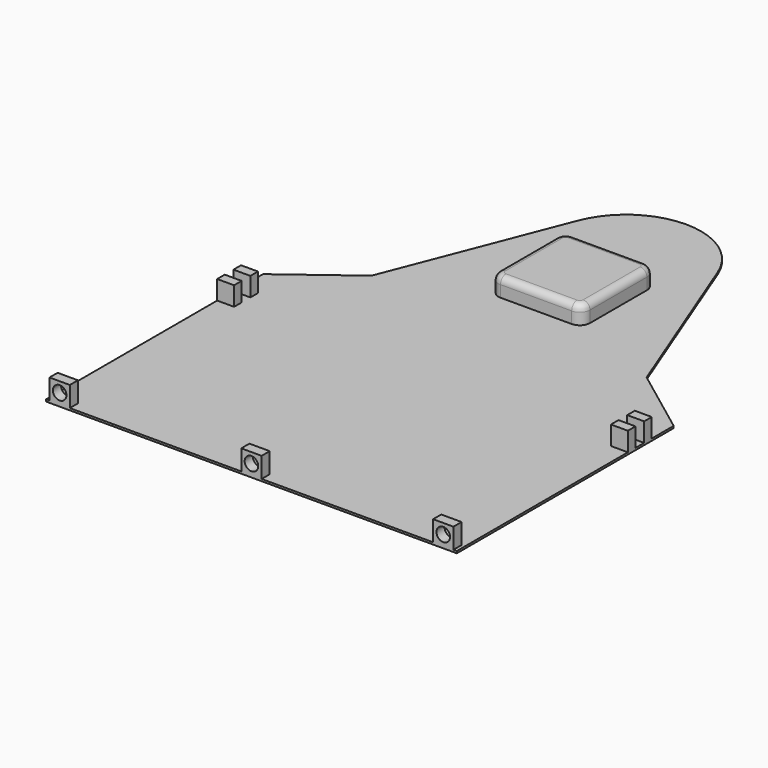
from build123d import *

# Parameters (mm, degrees)
F0_W         = 27
F0_H         = 27
F1_DEPTH     = 0.6
F2_DEPTH     = 6
F3_R         = 2
F4_T1_DEPTH  = 5.4
F4_T4_ANGLE  = 90
F4_T6_ANGLE  = 90
F4_T8_ANGLE  = 90
F4_T10_ANGLE = 90
F5_W         = 5
F5_H         = 2.8
F6_DEPTH     = 5.6
F7_W         = 6
F7_H         = 3
F8_DEPTH     = 6
F9_R         = 2
F10_DEPTH    = 4


# Not quite as in the source:
# - a fillet or chamfer that OpenCascade refuses, or shapes differently, is made with other operations: its cross-section is extruded or revolved along the edge and cut away or added


with BuildPart() as f1:
    # F0 (on Top) → F1 (new body)
    with BuildSketch(Plane.XY):
        with BuildLine():
            Line((-40.6, 95), (-60.6, 80))
            Line((-60.6, 80), (-60.6, 0))
            Line((-60.6, 0), (60.6, 0))
            Line((60.6, 0), (60.6, 80))
            Line((60.6, 80), (40.6, 95))
            Line((40.6, 95), (20.6, 146.2347538298))
            ThreePointArc((20.6, 146.2347538298), (0, 160.3072328817), (-20.6, 146.2347538298))
            Line((-20.6, 146.2347538298), (-40.6, 95))
        make_face()
        with Locations((0, 118.5)):
            Rectangle(F0_W, F0_H, mode=Mode.SUBTRACT)
        with Locations((0, 118.5)):
            Rectangle(F0_W, F0_H)
    extrude(amount=F1_DEPTH)

    # F0 (on Top) → F2 (join)
    with BuildSketch(Plane.XY):
        with Locations((0, 118.5)):
            Rectangle(F0_W, F0_H)
    extrude(amount=F2_DEPTH)

    # F3
    f3_edges = [f1.edges().sort_by_distance(p)[0] for p in [
        (0, 132, 6),
        (-13.5, 118.5, 6),
        (0, 105, 6),
        (13.5, 118.5, 6),
    ]]
    fillet(f3_edges, radius=F3_R)

    # F4: fillet of radius 3 on 4 edges, made by hand

    # F4_s2 → F4_t1 (cut)
    with BuildSketch(Plane.XY.offset(0.6)):
        with BuildLine():
            ThreePointArc((-13.5, 129), (-12.6213203436, 131.1213203436), (-10.5, 132))
            Line((-10.5, 132), (-13.5, 132))
            Line((-13.5, 132), (-13.5, 129))
        make_face()
        with BuildLine():
            ThreePointArc((-13.5, 108), (-12.6213203436, 105.8786796564), (-10.5, 105))
            Line((-10.5, 105), (-13.5, 105))
            Line((-13.5, 105), (-13.5, 108))
        make_face()
        with BuildLine():
            ThreePointArc((10.5, 105), (12.6213203436, 105.8786796564), (13.5, 108))
            Line((13.5, 108), (13.5, 105))
            Line((13.5, 105), (10.5, 105))
        make_face()
        with BuildLine():
            ThreePointArc((10.5, 132), (12.6213203436, 131.1213203436), (13.5, 129))
            Line((13.5, 129), (13.5, 132))
            Line((13.5, 132), (10.5, 132))
        make_face()
    extrude(amount=F4_T1_DEPTH, mode=Mode.SUBTRACT)

    # F4_s3 → F4_t4 (revolve, cut)
    with BuildSketch(Plane.XZ.offset(-129)):
        with BuildLine():
            ThreePointArc((11.5, 6), (12.9142135624, 5.4142135624), (13.5, 4))
            Line((13.5, 4), (13.5, 6))
            Line((13.5, 6), (11.5, 6))
        make_face()
    revolve(axis=Axis((10.5, 129, 6), (0, 0, 1)), revolution_arc=F4_T4_ANGLE, mode=Mode.SUBTRACT)

    # F4_s5 → F4_t6 (revolve, cut)
    with BuildSketch(Plane.YZ.offset(10.5)):
        with BuildLine():
            ThreePointArc((107, 6), (105.5857864376, 5.4142135624), (105, 4))
            Line((105, 4), (105, 6))
            Line((105, 6), (107, 6))
        make_face()
    revolve(axis=Axis((10.5, 108, 6), (0, 0, 1)), revolution_arc=F4_T6_ANGLE, mode=Mode.SUBTRACT)

    # F4_s7 → F4_t8 (revolve, cut)
    with BuildSketch(Plane.XZ.offset(-108)):
        with BuildLine():
            ThreePointArc((-11.5, 6), (-12.9142135624, 5.4142135624), (-13.5, 4))
            Line((-13.5, 4), (-13.5, 6))
            Line((-13.5, 6), (-11.5, 6))
        make_face()
    revolve(axis=Axis((-10.5, 108, 6), (0, 0, 1)), revolution_arc=F4_T8_ANGLE, mode=Mode.SUBTRACT)

    # F4_s9 → F4_t10 (revolve, cut)
    with BuildSketch(Plane.YZ.offset(-10.5)):
        with BuildLine():
            ThreePointArc((130, 6), (131.4142135624, 5.4142135624), (132, 4))
            Line((132, 4), (132, 6))
            Line((132, 6), (130, 6))
        make_face()
    revolve(axis=Axis((-10.5, 129, 6), (0, 0, 1)), revolution_arc=F4_T10_ANGLE, mode=Mode.SUBTRACT)

    # F5 (on face) → F6 (join)
    with BuildSketch(Plane.XY.offset(0.6)):
        with Locations((-58.1, 70.5)):
            Rectangle(F5_W, F5_H)
        with Locations((-58.1, 64.5)):
            Rectangle(F5_W, F5_H)
        with Locations((58.1, 70.5)):
            Rectangle(F5_W, F5_H)
        with Locations((58.1, 64.5)):
            Rectangle(F5_W, F5_H)
    extrude(amount=F6_DEPTH)

    # F7 (on face) → F8 (join)
    with BuildSketch(Plane.XY.offset(0.6)):
        with Locations((-56.6, 1.5)):
            Rectangle(F7_W, F7_H)
        with Locations((56.6, 1.5)):
            Rectangle(F7_W, F7_H)
        with Locations((0, 1.5)):
            Rectangle(F7_W, F7_H)
    extrude(amount=F8_DEPTH)

    # F9 (on face) → F10 (cut)
    with BuildSketch(Plane.XZ):
        with Locations((56.6, 3.6)):
            Circle(F9_R)
        with Locations((-56.6, 3.6)):
            Circle(F9_R)
        with Locations((0, 3.6)):
            Circle(F9_R)
    extrude(amount=-F10_DEPTH, mode=Mode.SUBTRACT)


solid = f1.part
